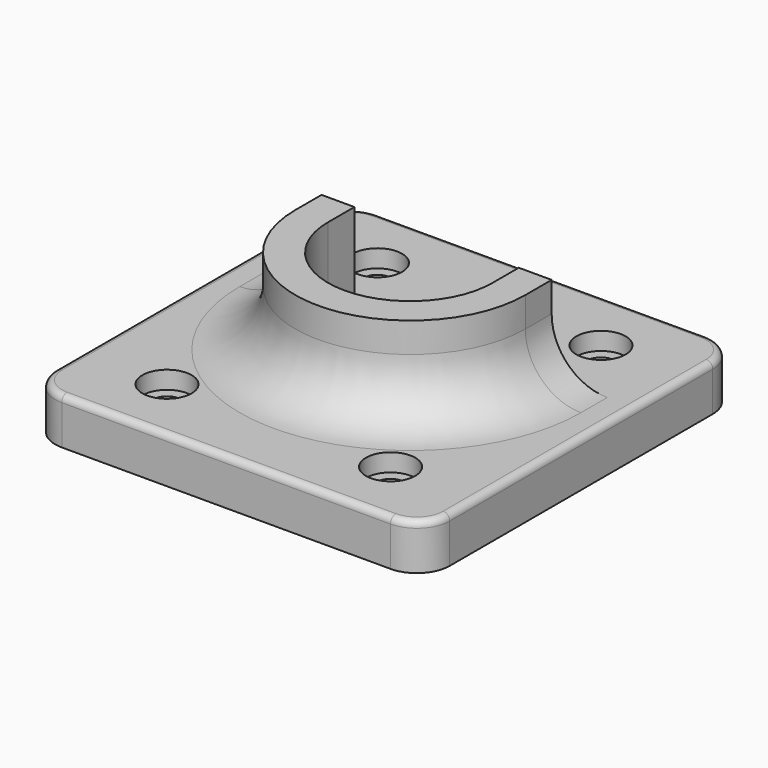
from build123d import *

# Parameters (mm, degrees)
F0_W     = 60
F0_H     = 60
F1_DEPTH = 7
F2_DEPTH = 20
F3_R     = 8.4497474683
F4_R     = 5
F5_R     = 1
F6_R     = 2.1
F7_DEPTH = 25
F6_R_2   = 3.75
F8_DEPTH = 2.7


# Not quite as in the source:
# - a feature names something its author has since deleted; it is built from what else it names


with BuildPart() as f1:
    # F0 (on Top) → F1 (new body)
    with BuildSketch(Plane.XY):
        Rectangle(F0_W, F0_H)
        with BuildLine():
            ThreePointArc((-16.7705098312, 10), (0, 22.5), (16.7705098312, 10))
            Line((16.7705098312, 10), (17.5, 10))
            Line((17.5, 10), (17.5, 5))
            ThreePointArc((17.5, 5), (0, -12.5), (-17.5, 5))
            Line((-17.5, 5), (-17.5, 10))
            Line((-17.5, 10), (-16.7705098312, 10))
        make_face(mode=Mode.SUBTRACT)
        with BuildLine():
            ThreePointArc((-12.5, 5), (0, -7.5), (12.5, 5))
            ThreePointArc((12.5, 5), (0, 17.5), (-12.5, 5))
        make_face()
        with BuildLine():
            ThreePointArc((-12.5, 5), (0, 17.5), (12.5, 5))
            Line((12.5, 5), (12.5, 10))
            Line((12.5, 10), (16.7705098312, 10))
            ThreePointArc((16.7705098312, 10), (0, 22.5), (-16.7705098312, 10))
            Line((-16.7705098312, 10), (-12.5, 10))
            Line((-12.5, 10), (-12.5, 5))
        make_face()
        with BuildLine():
            Line((12.5, 10), (12.5, 5))
            ThreePointArc((12.5, 5), (0, -7.5), (-12.5, 5))
            Line((-12.5, 5), (-12.5, 10))
            Line((-12.5, 10), (-16.7705098312, 10))
            ThreePointArc((-16.7705098312, 10), (-17.3166671454, 7.5264676876), (-17.5, 5))
            ThreePointArc((-17.5, 5), (0, -12.5), (17.5, 5))
            ThreePointArc((17.5, 5), (17.3166671454, 7.5264676876), (16.7705098312, 10))
            Line((16.7705098312, 10), (12.5, 10))
        make_face()
        with BuildLine():
            ThreePointArc((-17.5, 5), (-17.3166671454, 7.5264676876), (-16.7705098312, 10))
            Line((-16.7705098312, 10), (-17.5, 10))
            Line((-17.5, 10), (-17.5, 5))
        make_face()
        with BuildLine():
            Line((17.5, 10), (16.7705098312, 10))
            ThreePointArc((16.7705098312, 10), (17.3166671454, 7.5264676876), (17.5, 5))
            Line((17.5, 5), (17.5, 10))
        make_face()
    extrude(amount=F1_DEPTH)

    # F0 (on Top) → F2 (join)
    with BuildSketch(Plane.XY):
        with BuildLine():
            Line((12.5, 10), (12.5, 5))
            ThreePointArc((12.5, 5), (0, -7.5), (-12.5, 5))
            Line((-12.5, 5), (-12.5, 10))
            Line((-12.5, 10), (-16.7705098312, 10))
            ThreePointArc((-16.7705098312, 10), (-17.3166671454, 7.5264676876), (-17.5, 5))
            ThreePointArc((-17.5, 5), (0, -12.5), (17.5, 5))
            ThreePointArc((17.5, 5), (17.3166671454, 7.5264676876), (16.7705098312, 10))
            Line((16.7705098312, 10), (12.5, 10))
        make_face()
        with BuildLine():
            Line((17.5, 10), (16.7705098312, 10))
            ThreePointArc((16.7705098312, 10), (17.3166671454, 7.5264676876), (17.5, 5))
            Line((17.5, 5), (17.5, 10))
        make_face()
        with BuildLine():
            ThreePointArc((-17.5, 5), (-17.3166671454, 7.5264676876), (-16.7705098312, 10))
            Line((-16.7705098312, 10), (-17.5, 10))
            Line((-17.5, 10), (-17.5, 5))
        make_face()
    extrude(amount=F2_DEPTH)

    # F3
    f3_edges = [f1.edges().sort_by_distance(p)[0] for p in [
        (0, -12.5, 7),
        (-17.5, 7.5, 7),
        (17.5, 7.5, 7),
    ]]
    fillet(f3_edges, radius=F3_R)

    # F4
    f4_edges = [f1.edges().sort_by_distance(p)[0] for p in [
        (30, -30, 3.5),
        (-30, -30, 3.5),
        (-30, 30, 3.5),
        (30, 30, 3.5),
    ]]
    fillet(f4_edges, radius=F4_R)

    # F5
    f5_edges = [f1.edges().sort_by_distance(p)[0] for p in [
        (-30, 0, 7),
        (-28.535534, 28.535534, 7),
        (0, 30, 7),
        (30, 0, 7),
        (28.535534, 28.535534, 7),
        (0, -30, 7),
        (-28.535534, -28.535534, 7),
        (28.535534, -28.535534, 7),
    ]]
    fillet(f5_edges, radius=F5_R)

    # F6 (on face) → F7 (cut)
    with BuildSketch(Plane.XY.offset(7)):
        with Locations((-17, 20)):
            Circle(F6_R)
        with Locations((17, 20)):
            Circle(F6_R)
        with Locations((-17, -20)):
            Circle(F6_R)
        with Locations((17, -20)):
            Circle(F6_R)
    extrude(amount=-F7_DEPTH, mode=Mode.SUBTRACT)

    # F6 (on face) → F8 (cut)
    with BuildSketch(Plane.XY.offset(7)):
        with Locations((-17, 20)):
            Circle(F6_R_2)
        with Locations((-17, 20)):
            Circle(F6_R, mode=Mode.SUBTRACT)
        with Locations((17, 20)):
            Circle(F6_R_2)
        with Locations((17, 20)):
            Circle(F6_R, mode=Mode.SUBTRACT)
        with Locations((-17, -20)):
            Circle(F6_R_2)
        with Locations((-17, -20)):
            Circle(F6_R, mode=Mode.SUBTRACT)
        with Locations((17, -20)):
            Circle(F6_R_2)
        with Locations((17, -20)):
            Circle(F6_R, mode=Mode.SUBTRACT)
    extrude(amount=-F8_DEPTH, mode=Mode.SUBTRACT)


solid = f1.part
